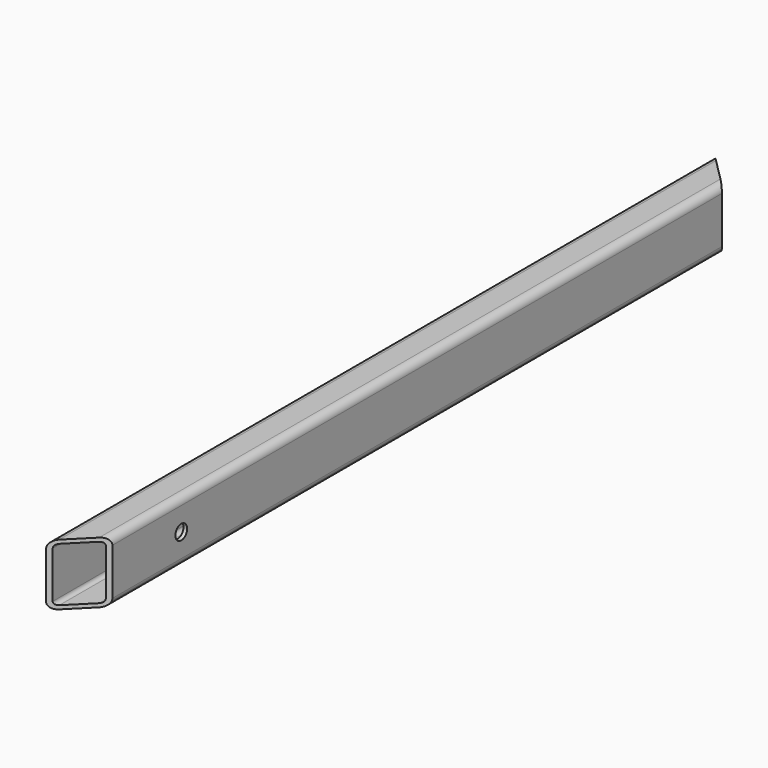
from build123d import *

# Parameters (mm, degrees)
F1_DEPTH = 340
F3_DEPTH = 50
F5_D     = 12


# Not quite as in the source:
# - a feature names something its author has since deleted; it is built from what else it names


with BuildPart() as f1:
    # F0 (on Front) → F1 (new body, symmetric)
    with BuildSketch(Plane.XZ):
        with BuildLine():
            ThreePointArc((15, 19), (13.2426406871, 23.2426406871), (9, 25))
            Line((9, 25), (-9, 25))
            ThreePointArc((-9, 25), (-13.2426406871, 23.2426406871), (-15, 19))
            Line((-15, 19), (-15, -19))
            ThreePointArc((-15, -19), (-13.2426406871, -23.2426406871), (-9, -25))
            Line((-9, -25), (9, -25))
            ThreePointArc((9, -25), (13.2426406871, -23.2426406871), (15, -19))
            Line((15, -19), (15, 19))
        make_face()
        with BuildLine():
            Line((-9, 22), (9, 22))
            ThreePointArc((9, 22), (11.1213203436, 21.1213203436), (12, 19))
            Line((12, 19), (12, -19))
            ThreePointArc((12, -19), (11.1213203436, -21.1213203436), (9, -22))
            Line((9, -22), (-9, -22))
            ThreePointArc((-9, -22), (-11.1213203436, -21.1213203436), (-12, -19))
            Line((-12, -19), (-12, 19))
            ThreePointArc((-12, 19), (-11.1213203436, 21.1213203436), (-9, 22))
        make_face(mode=Mode.SUBTRACT)
    extrude(amount=F1_DEPTH, both=True)

    # F2 (on face) → F3 (cut, through all)
    with BuildSketch(Plane.XY.offset(25)):
        Polygon((-9, -340), (-9, -334), (-15, -340), align=None)
        Polygon((9, -340), (9, -316), (-9, -334), (-9, -340), align=None)
        Polygon((15, -310), (9, -316), (9, -340), (15, -340), align=None)
        Polygon((-15, 340), (-9, 334), (-9, 340), align=None)
        Polygon((-9, 334), (9, 316), (9, 340), (-9, 340), align=None)
        Polygon((9, 316), (15, 310), (15, 340), (9, 340), align=None)
    extrude(amount=-F3_DEPTH, mode=Mode.SUBTRACT)

    # F5 (through all)
    with Locations(Plane(origin=(-15, 0, 0), x_dir=(0, -1, 0), z_dir=(-1, 0, 0))):
        with Locations((240, 0)):
            Hole(F5_D / 2)


solid = f1.part
